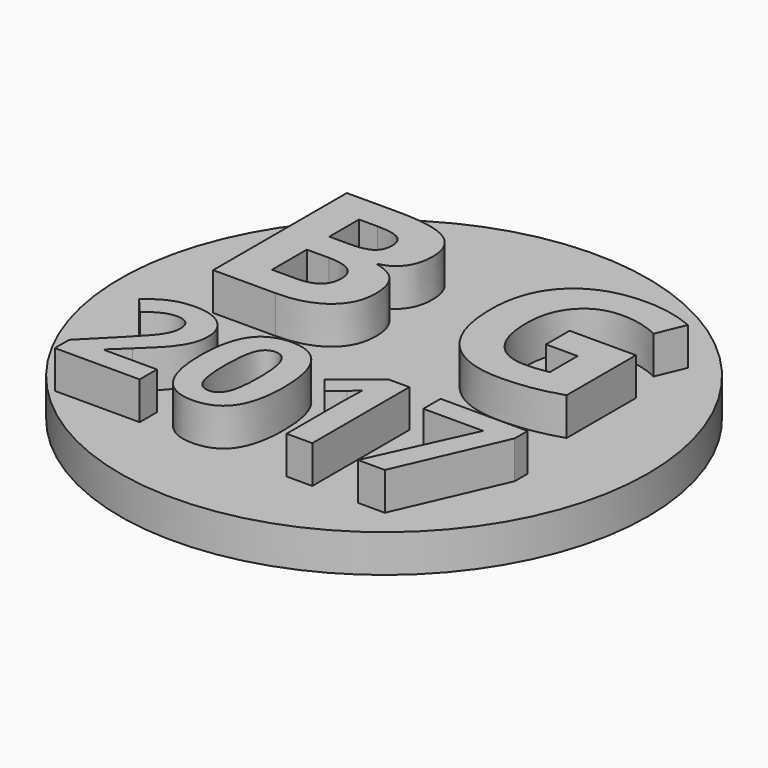
from build123d import *

# Parameters (mm, degrees)
F0_R           = 7
F1_DEPTH       = 1
F3_TEXT_SIZE   = 6.2045217155
F3_TEXT_SIZE_2 = 4.5072549661
F4_DEPTH       = 1


# Not quite as in the source:
# - Text() gives the source's letters only with a copy of the font that has no kerning and outlines rounded to 1/6400 em; it was checked with that copy


with BuildPart() as f1:
    # F0 (on Top) → F1 (new body)
    with BuildSketch(Plane.XY):
        Circle(F0_R)
    extrude(amount=F1_DEPTH)


with BuildPart() as f4:
    # F3 (on offset) → F4 (new body)
    with BuildSketch(Plane.XY.offset(1)):
        with Locations((-5.0896467197, 0)):
            Text('B G', F3_TEXT_SIZE, font='Open Sans', font_style=FontStyle.BOLD, text_align=(TextAlign.LEFT, TextAlign.BOTTOM))
        with Locations((-5.0896467197, -4.7775669083)):
            Text('2017', F3_TEXT_SIZE_2, font='Open Sans', font_style=FontStyle.BOLD, text_align=(TextAlign.LEFT, TextAlign.BOTTOM))
    extrude(amount=F4_DEPTH)


solid = Compound([f1.part, f4.part])
